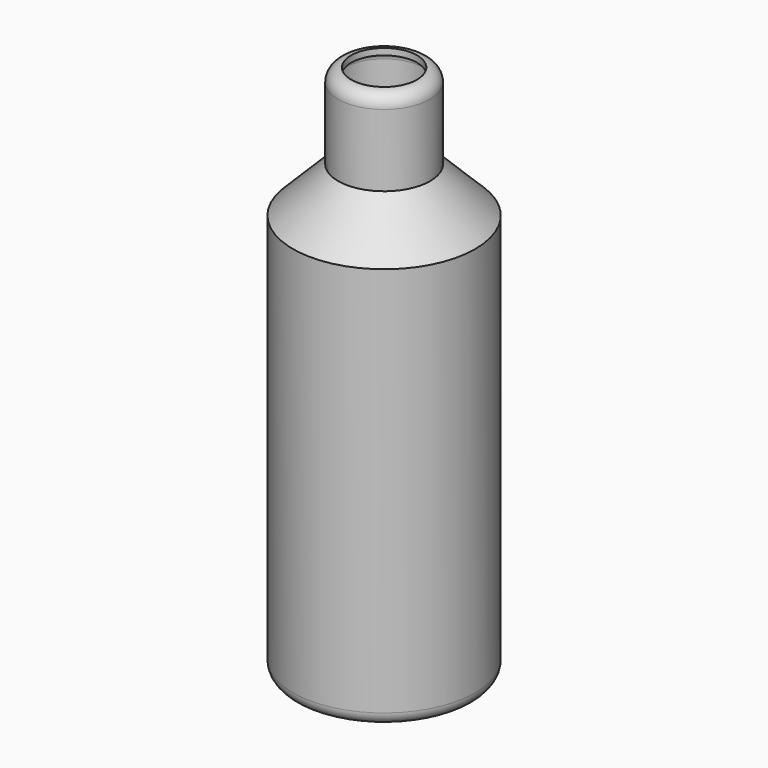
from build123d import *

# Parameters (mm, degrees)
F0_R        = 35
F1_DEPTH    = 180
F2_R        = 15
F3_DEPTH    = 10
F4_SIZE     = 4.99999
F5_R        = 17.6680128579
F6_DEPTH    = 25
F7_R        = 5
F8_R        = 5
F9_S5_R     = 17.6680128579
F9_T6_DEPTH = 53
F10_T       = 2.5


# Not quite as in the source:
# - a fillet or chamfer that OpenCascade refuses, or shapes differently, is made with other operations: its cross-section is extruded or revolved along the edge and cut away or added
# - a fillet or chamfer is up to 0.001 mm smaller than in the source, because OpenCascade refuses the exact size
# - a shell that OpenCascade refuses in one call is made with other operations: the cavity is built on its own and cut out


with BuildPart() as f1:
    # F0 (on Top) → F1 (new body)
    with BuildSketch(Plane.XY):
        Circle(F0_R)
    extrude(amount=F1_DEPTH)

    # F2 (on face) → F3 (cut)
    with BuildSketch(Plane(origin=(0, 0, 0), x_dir=(1, 0, 0), z_dir=(0, 0, -1))):
        Circle(F2_R)
    extrude(amount=-F3_DEPTH, mode=Mode.SUBTRACT)

    # F4 (size 5 in the source; OpenCascade refuses exactly that, so slightly less here)
    f4_edges = [f1.edges().sort_by_distance(p)[0] for p in [
        (-15, 0, 10),
        (-15, 0, 0),
    ]]
    chamfer(f4_edges, length=F4_SIZE)

    # F5 (on face) → F6 (join)
    with BuildSketch(Plane.XY.offset(180)):
        Circle(F5_R)
    extrude(amount=F6_DEPTH)

    # F7
    f7_edges = [f1.edges().sort_by_distance(p)[0] for p in [
        (-17.668013, 0, 205),
    ]]
    fillet(f7_edges, radius=F7_R)

    # F8
    f8_edges = [f1.edges().sort_by_distance(p)[0] for p in [
        (-35, 0, 0),
    ]]
    fillet(f8_edges, radius=F8_R)

    # F9: chamfer of 25 on 1 edges, made by hand


with BuildPart() as f9_tool2:
    # F9_s3 → F9_t4 (revolve)
    with BuildSketch(Plane.XZ):
        Polygon((35, 155), (10, 180), (35, 180), align=None)
    revolve(axis=Axis((0, 0, 180), (0, 0, 1)))

    # F9_s5 → F9_t6 (cut, symmetric)
    with BuildSketch(Plane.XY.offset(167.5)):
        Circle(F9_S5_R)
    extrude(amount=F9_T6_DEPTH, both=True, mode=Mode.SUBTRACT)


with BuildPart() as f1_1:
    add(f1.part)

    # F9_t1: cut F9_tool2
    add(f9_tool2.part, mode=Mode.SUBTRACT)

    # F10: shell of thickness 2.5, made by hand


with BuildPart() as f10_core1:
    # F10_t2: copy of F1
    add(f1_1.part)

    # the walls: a layer under each face that stays
    f10_faces = [f10_core1.faces().sort_by_distance(p)[0] for p in [
        (-35, 0, 80),
        (-26.334006429, 0, 163.665993571),
        (-17.6680128579, 0, 186.165993571),
        (-16.2035467638, 0, 203.5355339059),
        (-33.5355339059, 0, 1.4644660941),
        (-20, -20, 0),
        (-17.499995, 0, 2.499995),
        (-15, 0, 5),
        (-12.500005, 0, 7.500005),
        (0, 0, 10),
    ]]
    thicken(f10_faces, amount=-F10_T, mode=Mode.SUBTRACT)

    # F10_s3 → F10_t4 (revolve, cut)
    with BuildSketch(Plane.XZ):
        Polygon((17.7106905274, 172.3496648116), (15.9002459049, 170.5642201891), (15.1680128579, 171.2964532362), (15.1680128579, 172.3319871421), align=None)
    revolve(axis=Axis((0, 0, 172.3319871421), (0, 0, 1)), mode=Mode.SUBTRACT)

    # F10_s5 → F10_t6 (revolve, cut)
    with BuildSketch(Plane.XZ):
        Polygon((14.9573223305, 4.9823323305), (17.5, 5.00001), (17.5, 6.0355439059), (16.767766953, 6.767776953), align=None)
    revolve(axis=Axis((0, 0, 5.00001), (0, 0, -1)), mode=Mode.SUBTRACT)

    # F10_s7 → F10_t8 (revolve, cut)
    with BuildSketch(Plane.XZ):
        Polygon((9.9823323305, 9.9573223305), (11.767776953, 11.767766953), (11.0355439059, 12.5), (10.00001, 12.5), align=None)
    revolve(axis=Axis((0, 0, 10), (0, 0, -1)), mode=Mode.SUBTRACT)


with BuildPart() as f1_2:
    add(f1_1.part)

    # what is left inside the walls is the cavity
    f10_cavity = [f10_core1.part.solids().sort_by_distance(p)[0] for p in [
        (-32.475, 0, 104.309644),
    ]]
    add(f10_cavity, mode=Mode.SUBTRACT)


solid = f1_2.part
